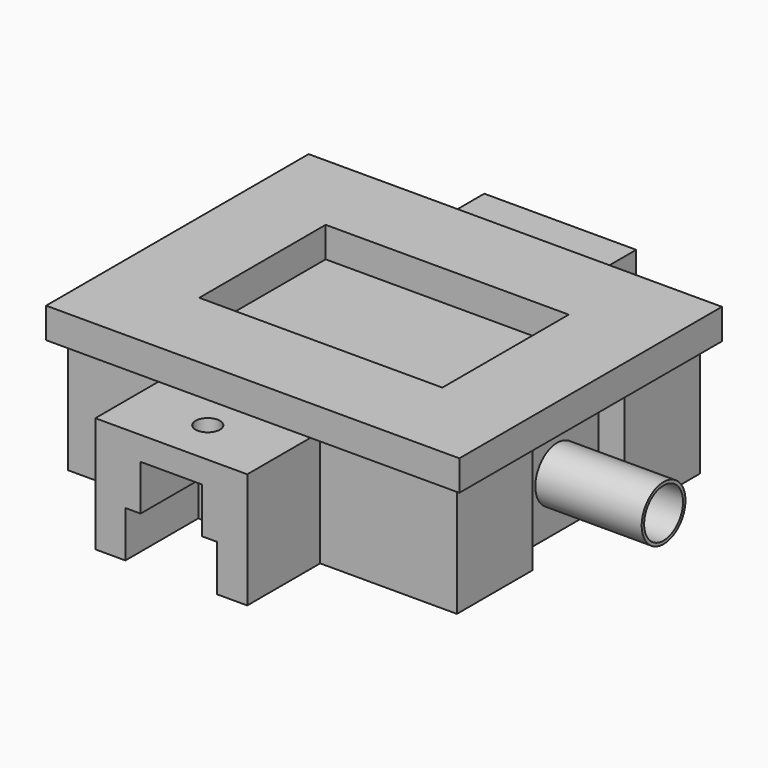
from build123d import *

# Parameters (mm, degrees)
F0_W      = 54
F0_H      = 19
F1_DEPTH  = 20
F2_R      = 4.5
F3_DEPTH  = 1.5
F4_DEPTH  = 19
F5_T      = -0.5
F6_W      = 64
F6_H      = 50
F6_W_2    = 54
F6_H_2    = 40
F7_DEPTH  = 19
F9_DEPTH  = 25
F10_W     = 68
F10_H     = 54
F10_W_2   = 64
F10_H_2   = 50
F11_DEPTH = 5
F10_W_3   = 54
F10_H_3   = 40
F10_W_4   = 40
F10_H_4   = 26
F14_DEPTH = 15
F15_R     = 2
F16_DEPTH = 8.901


with BuildPart() as f1:
    # F0 (on Front) → F1 (new body, symmetric)
    with BuildSketch(Plane.XZ):
        with Locations((3, 9.5)):
            Rectangle(F0_W, F0_H)
    extrude(amount=F1_DEPTH, both=True)

    # F2 (on face) → F3 (join)
    with BuildSketch(Plane.YZ.offset(30)):
        Polygon((-8.5, 17.5), (-8.5, 0.5), (0, 0.5), (8.5, 0.5), (8.5, 17.5), (0, 17.5), align=None)
        with Locations((0, 9)):
            Circle(F2_R, mode=Mode.SUBTRACT)
    extrude(amount=F3_DEPTH)

    # F4 (add): a face of the model
    f4_faces = [f1.faces().sort_by_distance(p)[0] for p in [
        (30, 0, 9),
    ]]
    extrude(f4_faces, amount=F4_DEPTH)

    # F5
    f5_openings = [f1.faces().sort_by_distance(p)[0] for p in [
        (49, 0, 9),
    ]]
    offset(amount=F5_T, openings=f5_openings, kind=Kind.INTERSECTION)


with BuildPart() as f7:
    # F6 (on face) → F7 (new body, through all)
    with BuildSketch(Plane.XY.offset(19)):
        with Locations((3, 0)):
            Rectangle(F6_W, F6_H)
        with Locations((3, 0)):
            Rectangle(F6_W_2, F6_H_2, mode=Mode.SUBTRACT)
    extrude(amount=-F7_DEPTH)

    # F8 (on face) → F9 (cut)
    with BuildSketch(Plane.YZ.offset(35)):
        Polygon((0, -0.5), (9.5, -0.5), (9.5, 19), (0, 19), (-9.5, 19), (-9.5, -0.5), align=None)
    extrude(amount=-F9_DEPTH, mode=Mode.SUBTRACT)

    # F12 (on face) → F14 (join)
    with BuildSketch(Plane(origin=(0, 25, 0), x_dir=(-1, 0, 0), z_dir=(0, 1, 0))):
        Polygon((-12.5, 0), (-7.55, 0), (-7.55, 7.6), (-5.05, 7.6), (-5.05, 15.1), (0, 15.1), (5.05, 15.1), (5.05, 7.6), (7.55, 7.6), (7.55, 0), (12.5, 0), (12.5, 19), (0, 19), (-12.5, 19), align=None)
    extrude(amount=F14_DEPTH)

    # F15 (on face) → F16 (cut, through all)
    with BuildSketch(Plane(origin=(0, 0, 15.1), x_dir=(1, 0, 0), z_dir=(0, 0, -1))):
        with Locations((0, -32.5)):
            Circle(F15_R)
    extrude(amount=-F16_DEPTH, mode=Mode.SUBTRACT)

    # F17: F7 across plane


with BuildPart() as f11:
    # F10 (on face) → F11 (new body)
    with BuildSketch(Plane.XY.offset(19)):
        with Locations((3, 0)):
            Rectangle(F10_W, F10_H)
        with Locations((3, 0)):
            Rectangle(F10_W_2, F10_H_2, mode=Mode.SUBTRACT)
    extrude(amount=F11_DEPTH)



with BuildPart() as f11b:
    # F10 (on face) → F11, piece 2 (new body)
    with BuildSketch(Plane.XY.offset(19)):
        with Locations((3, 0)):
            Rectangle(F10_W_3, F10_H_3)
        with Locations((3, 0)):
            Rectangle(F10_W_4, F10_H_4, mode=Mode.SUBTRACT)
    extrude(amount=F11_DEPTH)


with BuildPart() as f11_1:
    add(f11.part)

    add(f11b.part)  # F11#3 merges F11b
    # F6 (on face) → F11, piece 3 (join)
    with BuildSketch(Plane.XY.offset(19)):
        with Locations((3, 0)):
            Rectangle(F6_W, F6_H)
        with Locations((3, 0)):
            Rectangle(F6_W_2, F6_H_2, mode=Mode.SUBTRACT)
    extrude(amount=F11_DEPTH)


with BuildPart() as f7_1:
    add(f7.part)
    add(f7.part.mirror(Plane.XZ))


solid = Compound([f1.part, f11_1.part, f7_1.part])
